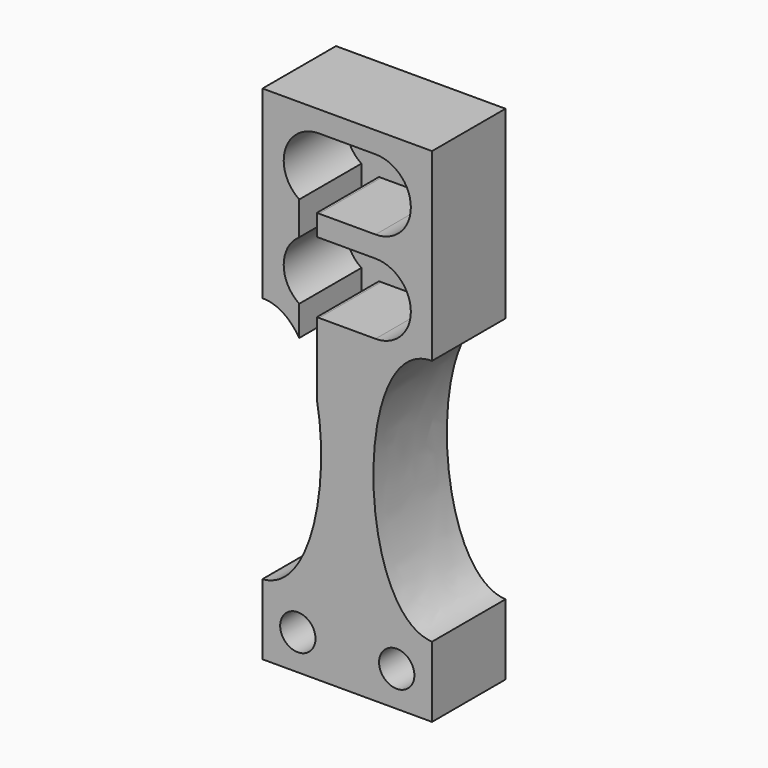
from build123d import *

# Parameters (mm, degrees)
F0_R     = 3.175
F1_DEPTH = 16.51
F2_DEPTH = 2.54


# Not quite as in the source:
# - a feature names something its author has since deleted; it is built from what else it names


with BuildPart() as f1:
    # F0 (on Front) → F1 (new body)
    with BuildSketch(Plane.XZ):
        with BuildLine():
            Line((15.24, 10.16), (0, 10.16))
            Line((0, 10.16), (-15.24, 10.16))
            Line((-15.24, 10.16), (-15.24, -23.0504914403))
            add(Edge.make_bspline(
                [(-15.24, -23.0504914403), (-12.4936951429, -23.050233708), (-10.2976989889, -24.6278435924), (-8.636, -27.1888607202)],
                knots=[0, 0, 0, 0, 8.4526904957, 8.4526904957, 8.4526904957, 8.4526904957], degree=3))
            Line((-8.636, -27.1888607202), (-8.636, -21.770928055))
            ThreePointArc((-8.636, -21.770928055), (-11.43, -16.51), (-8.636, -11.249071945))
            Line((-8.636, -11.249071945), (-8.636, -5.260928055))
            ThreePointArc((-8.636, -5.260928055), (-11.1516304709, 1.8595169871), (-5.08, 6.35))
            Line((-5.08, 6.35), (5.08, 6.35))
            ThreePointArc((5.08, 6.35), (9.5701280605, 4.4901280605), (11.43, 0))
            ThreePointArc((11.43, 0), (9.5701280605, -4.4901280605), (5.08, -6.35))
            Line((5.08, -6.35), (-5.08, -6.35))
            ThreePointArc((-5.08, -6.35), (-5.2705858603, -6.3471392792), (-5.461, -6.3385596944))
            Line((-5.461, -6.3385596944), (-5.461, -10.1714403056))
            ThreePointArc((-5.461, -10.1714403056), (-5.2705858603, -10.1628607208), (-5.08, -10.16))
            Line((-5.08, -10.16), (5.08, -10.16))
            ThreePointArc((5.08, -10.16), (9.5701280605, -12.0198719395), (11.43, -16.51))
            ThreePointArc((11.43, -16.51), (9.5701280605, -21.0001280605), (5.08, -22.86))
            Line((5.08, -22.86), (-5.08, -22.86))
            ThreePointArc((-5.08, -22.86), (-5.2705858603, -22.8571392792), (-5.461, -22.8485596944))
            Line((-5.461, -22.8485596944), (-5.461, -35.926681818))
            add(Edge.make_bspline(
                [(-5.461, -35.926681818), (-3.0177559473, -48.8656738837), (-6.4817336355, -66.9757324356), (-15.24, -67.5004914403)],
                knots=[15.9624587288, 15.9624587288, 15.9624587288, 15.9624587288, 44.45, 44.45, 44.45, 44.45], degree=3))
            Line((-15.24, -67.5004914403), (-15.24, -80.2004914403))
            Line((-15.24, -80.2004914403), (0, -80.2004914403))
            Line((0, -80.2004914403), (15.24, -80.2004914403))
            Line((15.24, -80.2004914403), (15.24, -67.5004914403))
            add(Edge.make_bspline(
                [(15.24, -23.0504914403), (0.7980597731, -23.0491361081), (1.5742035665, -66.6816935827), (15.24, -67.5004914403)],
                knots=[0, 0, 0, 0, 44.45, 44.45, 44.45, 44.45], degree=3))
            Line((15.24, -23.0504914403), (15.24, 10.16))
        make_face()
        with Locations((-8.89, -73.8504914403)):
            Circle(F0_R, mode=Mode.SUBTRACT)
        with Locations((8.89, -73.8504914403)):
            Circle(F0_R, mode=Mode.SUBTRACT)
    extrude(amount=F1_DEPTH)

    # F0 (on Front) → F2 (join)
    with BuildSketch(Plane.XZ):
        with BuildLine():
            ThreePointArc((-5.08, 6.35), (-11.1516304709, 1.8595169871), (-8.636, -5.260928055))
            ThreePointArc((-8.636, -5.260928055), (-7.1209102718, -6.0130845048), (-5.461, -6.3385596944))
            ThreePointArc((-5.461, -6.3385596944), (-5.2705858603, -6.3471392792), (-5.08, -6.35))
            ThreePointArc((-5.08, -6.35), (-2.2401936686, -5.6796126628), (0, -3.81))
            ThreePointArc((0, -3.81), (-1.27, 0), (0, 3.81))
            ThreePointArc((0, 3.81), (-2.2401936686, 5.6796126628), (-5.08, 6.35))
        make_face()
        with BuildLine():
            ThreePointArc((5.08, 6.35), (2.2401936686, 5.6796126628), (0, 3.81))
            ThreePointArc((0, 3.81), (0.9441389426, 2.0080463142), (1.27, 0))
            ThreePointArc((1.27, 0), (0.9441389426, -2.0080463142), (0, -3.81))
            ThreePointArc((0, -3.81), (2.2401936686, -5.6796126628), (5.08, -6.35))
            ThreePointArc((5.08, -6.35), (9.5701280605, -4.4901280605), (11.43, 0))
            ThreePointArc((11.43, 0), (9.5701280605, 4.4901280605), (5.08, 6.35))
        make_face()
        with BuildLine():
            Line((5.08, 6.35), (-5.08, 6.35))
            ThreePointArc((-5.08, 6.35), (-2.2401936686, 5.6796126628), (0, 3.81))
            ThreePointArc((0, 3.81), (2.2401936686, 5.6796126628), (5.08, 6.35))
        make_face()
        with BuildLine():
            ThreePointArc((1.27, 0), (0.9441389426, 2.0080463142), (0, 3.81))
            ThreePointArc((0, 3.81), (-1.27, 0), (0, -3.81))
            ThreePointArc((0, -3.81), (0.9441389426, -2.0080463142), (1.27, 0))
        make_face()
        with BuildLine():
            ThreePointArc((0, -3.81), (-2.2401936686, -5.6796126628), (-5.08, -6.35))
            Line((-5.08, -6.35), (5.08, -6.35))
            ThreePointArc((5.08, -6.35), (2.2401936686, -5.6796126628), (0, -3.81))
        make_face()
        with BuildLine():
            Line((-5.461, -22.5981636269), (-5.461, -22.8485596944))
            ThreePointArc((-5.461, -22.8485596944), (-5.2705858603, -22.8571392792), (-5.08, -22.86))
            ThreePointArc((-5.08, -22.86), (-2.2401936686, -22.1896126628), (0, -20.32))
            ThreePointArc((0, -20.32), (-1.27, -16.51), (0, -12.7))
            ThreePointArc((0, -12.7), (-2.2401936686, -10.8303873372), (-5.08, -10.16))
            ThreePointArc((-5.08, -10.16), (-5.2705858603, -10.1628607208), (-5.461, -10.1714403056))
            Line((-5.461, -10.1714403056), (-5.461, -22.5981636269))
        make_face()
        with BuildLine():
            ThreePointArc((0, -12.7), (-1.27, -16.51), (0, -20.32))
            ThreePointArc((0, -20.32), (0.9441389426, -18.5180463142), (1.27, -16.51))
            ThreePointArc((1.27, -16.51), (0.9441389426, -14.5019536858), (0, -12.7))
        make_face()
        with BuildLine():
            Line((5.08, -10.16), (-5.08, -10.16))
            ThreePointArc((-5.08, -10.16), (-2.2401936686, -10.8303873372), (0, -12.7))
            ThreePointArc((0, -12.7), (2.2401936686, -10.8303873372), (5.08, -10.16))
        make_face()
        with BuildLine():
            ThreePointArc((1.27, -16.51), (0.9441389426, -18.5180463142), (0, -20.32))
            ThreePointArc((0, -20.32), (2.2401936686, -22.1896126628), (5.08, -22.86))
            ThreePointArc((5.08, -22.86), (9.5701280605, -21.0001280605), (11.43, -16.51))
            ThreePointArc((11.43, -16.51), (9.5701280605, -12.0198719395), (5.08, -10.16))
            ThreePointArc((5.08, -10.16), (2.2401936686, -10.8303873372), (0, -12.7))
            ThreePointArc((0, -12.7), (0.9441389426, -14.5019536858), (1.27, -16.51))
        make_face()
        with BuildLine():
            ThreePointArc((0, -20.32), (-2.2401936686, -22.1896126628), (-5.08, -22.86))
            Line((-5.08, -22.86), (5.08, -22.86))
            ThreePointArc((5.08, -22.86), (2.2401936686, -22.1896126628), (0, -20.32))
        make_face()
        with BuildLine():
            Line((-8.636, -21.770928055), (-8.636, -27.1888607202))
            add(Edge.make_bspline(
                [(-8.636, -27.1888607202), (-7.1596683768, -29.4641889225), (-6.1050779286, -32.5157580511), (-5.461, -35.926681818)],
                knots=[8.4526904957, 8.4526904957, 8.4526904957, 8.4526904957, 15.9624587288, 15.9624587288, 15.9624587288, 15.9624587288], degree=3))
            Line((-5.461, -35.926681818), (-5.461, -22.8485596944))
            ThreePointArc((-5.461, -22.8485596944), (-7.1209102718, -22.5230845048), (-8.636, -21.770928055))
        make_face()
        with BuildLine():
            Line((-8.636, -5.260928055), (-8.636, -11.249071945))
            ThreePointArc((-8.636, -11.249071945), (-7.1209102718, -10.4969154952), (-5.461, -10.1714403056))
            Line((-5.461, -10.1714403056), (-5.461, -6.3385596944))
            ThreePointArc((-5.461, -6.3385596944), (-7.1209102718, -6.0130845048), (-8.636, -5.260928055))
        make_face()
        with BuildLine():
            ThreePointArc((-8.636, -11.249071945), (-11.43, -16.51), (-8.636, -21.770928055))
            ThreePointArc((-8.636, -21.770928055), (-7.1209102718, -22.5230845048), (-5.461, -22.8485596944))
            Line((-5.461, -22.8485596944), (-5.461, -22.5981636269))
            Line((-5.461, -22.5981636269), (-5.461, -10.1714403056))
            ThreePointArc((-5.461, -10.1714403056), (-7.1209102718, -10.4969154952), (-8.636, -11.249071945))
        make_face()
    extrude(amount=F2_DEPTH)


solid = f1.part
